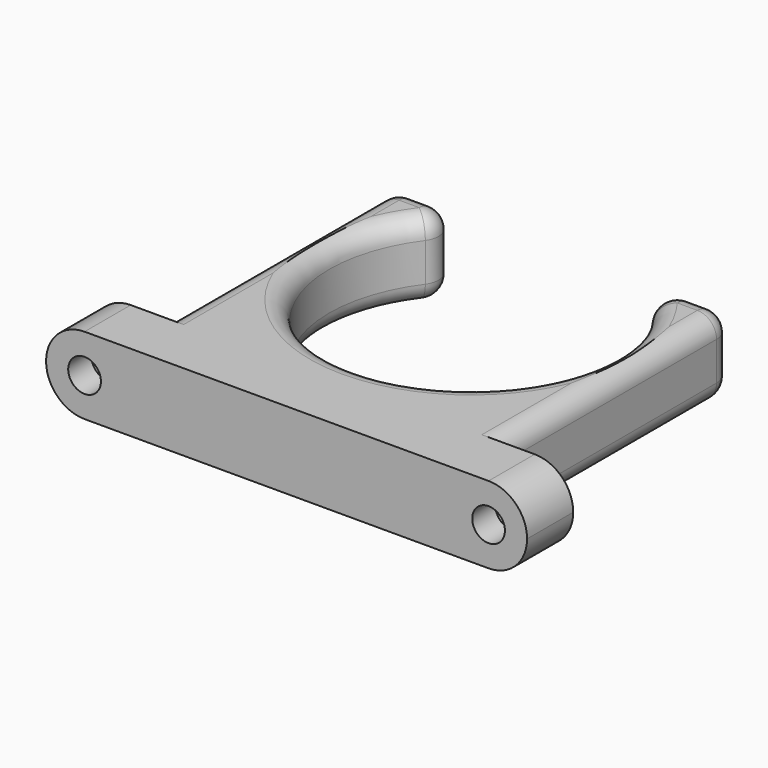
from build123d import *

# Parameters (mm, degrees)
F1_DEPTH             = 8
F4_D                 = 3.4
F4_CBORE_D           = 6.5
F4_CBORE_DEPTH       = 3
F4_ON_F3_D           = 3.4
F4_ON_F3_CBORE_D     = 6.5
F4_ON_F3_CBORE_DEPTH = 3
F5_T1_DEPTH          = 2.0779215299
F5_T3_DEPTH          = 28
F5_T5_DEPTH          = 2.0779215299
F5_T8_ANGLE          = 253.4876833877
F5_T10_ANGLE         = 253.4876833877
F5_T12_ANGLE         = 126.7438416939
F5_T14_ANGLE         = 126.7438416939
F5_T16_ANGLE         = 90
F5_T18_ANGLE         = 90
F5_T20_ANGLE         = 126.7438416939
F5_T22_ANGLE         = 126.7438416939
F5_T24_ANGLE         = 90
F5_T26_ANGLE         = 90
F6_R                 = 3.99999


# Not quite as in the source:
# - a fillet or chamfer that OpenCascade refuses, or shapes differently, is made with other operations: its cross-section is extruded or revolved along the edge and cut away or added
# - a fillet or chamfer is up to 0.001 mm smaller than in the source, because OpenCascade refuses the exact size


with BuildPart() as f1:
    # F0 (on Top) → F1 (new body)
    with BuildSketch(Plane.XY):
        Polygon((-25, 6), (-25, 0), (25, 0), (25, 6), (17.5, 6), (-17.5, 6), align=None)
        with BuildLine():
            Line((-17.5, 34), (-17.5, 6))
            Line((-17.5, 6), (17.5, 6))
            Line((17.5, 6), (17.5, 34))
            ThreePointArc((17.5, 34), (16.9142135624, 35.4142135624), (15.5, 36))
            Line((15.5, 36), (13.4220784701, 36))
            ThreePointArc((13.4220784701, 36), (11.634209081, 34.896394471), (11.8194422349, 32.8035230476))
            ThreePointArc((11.8194422349, 32.8035230476), (0, 9.229505524), (-11.8194422349, 32.8035230476))
            ThreePointArc((-11.8194422349, 32.8035230476), (-11.634209081, 34.896394471), (-13.4220784701, 36))
            Line((-13.4220784701, 36), (-15.5, 36))
            ThreePointArc((-15.5, 36), (-16.9142135624, 35.4142135624), (-17.5, 34))
        make_face()
    extrude(amount=F1_DEPTH)

    # F4 (through all)
    with Locations(Plane(origin=(0, 6, 0), x_dir=(-1, 0, 0), z_dir=(0, 1, 0))):
        with Locations((-21, 4)):
            CounterBoreHole(F4_D / 2, F4_CBORE_D / 2, F4_CBORE_DEPTH)

    # F4 on F3 (through all)
    with Locations(Plane(origin=(0, 6, 0), x_dir=(-1, 0, 0), z_dir=(0, 1, 0))):
        with Locations((21, 4)):
            CounterBoreHole(F4_ON_F3_D / 2, F4_ON_F3_CBORE_D / 2, F4_ON_F3_CBORE_DEPTH)

    # F5: fillet of radius 2 on 2 edges, made by hand

    # F5_s2 → F5_t1 (cut)
    with BuildSketch(Plane.YZ.offset(-15.5)):
        with BuildLine():
            ThreePointArc((34, 8), (35.4142135624, 7.4142135624), (36, 6))
            Line((36, 6), (36, 8))
            Line((36, 8), (34, 8))
        make_face()
        with BuildLine():
            ThreePointArc((34, 0), (35.4142135624, 0.5857864376), (36, 2))
            Line((36, 2), (36, 0))
            Line((36, 0), (34, 0))
        make_face()
    extrude(amount=F5_T1_DEPTH, mode=Mode.SUBTRACT)

    # F5_s4 → F5_t3 (cut)
    with BuildSketch(Plane.XZ.offset(-34)):
        with BuildLine():
            ThreePointArc((-15.5, 8), (-16.9142135624, 7.4142135624), (-17.5, 6))
            Line((-17.5, 6), (-17.5, 8))
            Line((-17.5, 8), (-15.5, 8))
        make_face()
        with BuildLine():
            ThreePointArc((15.5, 8), (16.9142135624, 7.4142135624), (17.5, 6))
            Line((17.5, 6), (17.5, 8))
            Line((17.5, 8), (15.5, 8))
        make_face()
        with BuildLine():
            ThreePointArc((-15.5, 0), (-16.9142135624, 0.5857864376), (-17.5, 2))
            Line((-17.5, 2), (-17.5, 0))
            Line((-17.5, 0), (-15.5, 0))
        make_face()
        with BuildLine():
            ThreePointArc((15.5, 0), (16.9142135624, 0.5857864376), (17.5, 2))
            Line((17.5, 2), (17.5, 0))
            Line((17.5, 0), (15.5, 0))
        make_face()
    extrude(amount=F5_T3_DEPTH, mode=Mode.SUBTRACT)

    # F5_s6 → F5_t5 (cut)
    with BuildSketch(Plane.YZ.offset(13.4220784701)):
        with BuildLine():
            ThreePointArc((34, 8), (35.4142135624, 7.4142135624), (36, 6))
            Line((36, 6), (36, 8))
            Line((36, 8), (34, 8))
        make_face()
        with BuildLine():
            ThreePointArc((34, 0), (35.4142135624, 0.5857864376), (36, 2))
            Line((36, 2), (36, 0))
            Line((36, 0), (34, 0))
        make_face()
    extrude(amount=F5_T5_DEPTH, mode=Mode.SUBTRACT)

    # F5_s7 → F5_t8 (revolve, cut)
    with BuildSketch(Plane(origin=(-11.4952792826, 15.3974976921, 0), x_dir=(0, 0, 1), z_dir=(-0.5982384762, 0.8013181176, 0))):
        with BuildLine():
            ThreePointArc((0, 31.0954628442), (0.5857864376, 29.6812492818), (2, 29.0954628442))
            Line((2, 29.0954628442), (0, 29.0954628442))
            Line((0, 29.0954628442), (0, 31.0954628442))
        make_face()
    revolve(axis=Axis((0, 23.979505524, 0), (0, 0, -1)), revolution_arc=F5_T8_ANGLE, mode=Mode.SUBTRACT)

    # F5_s9 → F5_t10 (revolve, cut)
    with BuildSketch(Plane(origin=(-11.4952792826, 15.3974976921, 0), x_dir=(0, 0, 1), z_dir=(-0.5982384762, 0.8013181176, 0))):
        with BuildLine():
            ThreePointArc((8, 31.0954628442), (7.4142135624, 29.6812492818), (6, 29.0954628442))
            Line((6, 29.0954628442), (8, 29.0954628442))
            Line((8, 29.0954628442), (8, 31.0954628442))
        make_face()
    revolve(axis=Axis((0, 23.979505524, 8), (0, 0, -1)), revolution_arc=F5_T10_ANGLE, mode=Mode.SUBTRACT)

    # F5_s11 → F5_t12 (revolve, cut)
    with BuildSketch(Plane.YZ.offset(13.4220784701)):
        with BuildLine():
            ThreePointArc((34, 8), (35.4142135624, 7.4142135624), (36, 6))
            Line((36, 6), (36, 8))
            Line((36, 8), (34, 8))
        make_face()
    revolve(axis=Axis((13.4220784701, 34, 8), (0, 0, 1)), revolution_arc=F5_T12_ANGLE, mode=Mode.SUBTRACT)

    # F5_s13 → F5_t14 (revolve, cut)
    with BuildSketch(Plane(origin=(11.4952792826, 15.3974976921, 0), x_dir=(0, 0, 1), z_dir=(-0.5982384762, -0.8013181176, 0))):
        with BuildLine():
            ThreePointArc((8, 31.0954628442), (7.4142135624, 29.6812492818), (6, 29.0954628442))
            Line((6, 29.0954628442), (8, 29.0954628442))
            Line((8, 29.0954628442), (8, 31.0954628442))
        make_face()
    revolve(axis=Axis((-13.4220784701, 34, 8), (0, 0, 1)), revolution_arc=F5_T14_ANGLE, mode=Mode.SUBTRACT)

    # F5_s15 → F5_t16 (revolve, cut)
    with BuildSketch(Plane.YZ.offset(-15.5)):
        with BuildLine():
            ThreePointArc((34, 8), (35.4142135624, 7.4142135624), (36, 6))
            Line((36, 6), (36, 8))
            Line((36, 8), (34, 8))
        make_face()
    revolve(axis=Axis((-15.5, 34, 8), (0, 0, 1)), revolution_arc=F5_T16_ANGLE, mode=Mode.SUBTRACT)

    # F5_s17 → F5_t18 (revolve, cut)
    with BuildSketch(Plane.XZ.offset(-34)):
        with BuildLine():
            ThreePointArc((15.5, 8), (16.9142135624, 7.4142135624), (17.5, 6))
            Line((17.5, 6), (17.5, 8))
            Line((17.5, 8), (15.5, 8))
        make_face()
    revolve(axis=Axis((15.5, 34, 8), (0, 0, 1)), revolution_arc=F5_T18_ANGLE, mode=Mode.SUBTRACT)

    # F5_s19 → F5_t20 (revolve, cut)
    with BuildSketch(Plane.YZ.offset(13.4220784701)):
        with BuildLine():
            ThreePointArc((34, 0), (35.4142135624, 0.5857864376), (36, 2))
            Line((36, 2), (36, 0))
            Line((36, 0), (34, 0))
        make_face()
    revolve(axis=Axis((13.4220784701, 34, 0), (0, 0, 1)), revolution_arc=F5_T20_ANGLE, mode=Mode.SUBTRACT)

    # F5_s21 → F5_t22 (revolve, cut)
    with BuildSketch(Plane(origin=(11.4952792826, 15.3974976921, 0), x_dir=(0, 0, 1), z_dir=(-0.5982384762, -0.8013181176, 0))):
        with BuildLine():
            ThreePointArc((0, 31.0954628442), (0.5857864376, 29.6812492818), (2, 29.0954628442))
            Line((2, 29.0954628442), (0, 29.0954628442))
            Line((0, 29.0954628442), (0, 31.0954628442))
        make_face()
    revolve(axis=Axis((-13.4220784701, 34, 0), (0, 0, 1)), revolution_arc=F5_T22_ANGLE, mode=Mode.SUBTRACT)

    # F5_s23 → F5_t24 (revolve, cut)
    with BuildSketch(Plane.YZ.offset(-15.5)):
        with BuildLine():
            ThreePointArc((34, 0), (35.4142135624, 0.5857864376), (36, 2))
            Line((36, 2), (36, 0))
            Line((36, 0), (34, 0))
        make_face()
    revolve(axis=Axis((-15.5, 34, 0), (0, 0, 1)), revolution_arc=F5_T24_ANGLE, mode=Mode.SUBTRACT)

    # F5_s25 → F5_t26 (revolve, cut)
    with BuildSketch(Plane.XZ.offset(-34)):
        with BuildLine():
            ThreePointArc((15.5, 0), (16.9142135624, 0.5857864376), (17.5, 2))
            Line((17.5, 2), (17.5, 0))
            Line((17.5, 0), (15.5, 0))
        make_face()
    revolve(axis=Axis((15.5, 34, 0), (0, 0, 1)), revolution_arc=F5_T26_ANGLE, mode=Mode.SUBTRACT)

    # F6 (radius 4 in the source; OpenCascade refuses exactly that, so slightly less here)
    f6_edges = [f1.edges().sort_by_distance(p)[0] for p in [
        (-25, 3, 0),
        (-25, 3, 8),
        (25, 3, 0),
        (25, 3, 8),
    ]]
    fillet(f6_edges, radius=F6_R)


solid = f1.part
